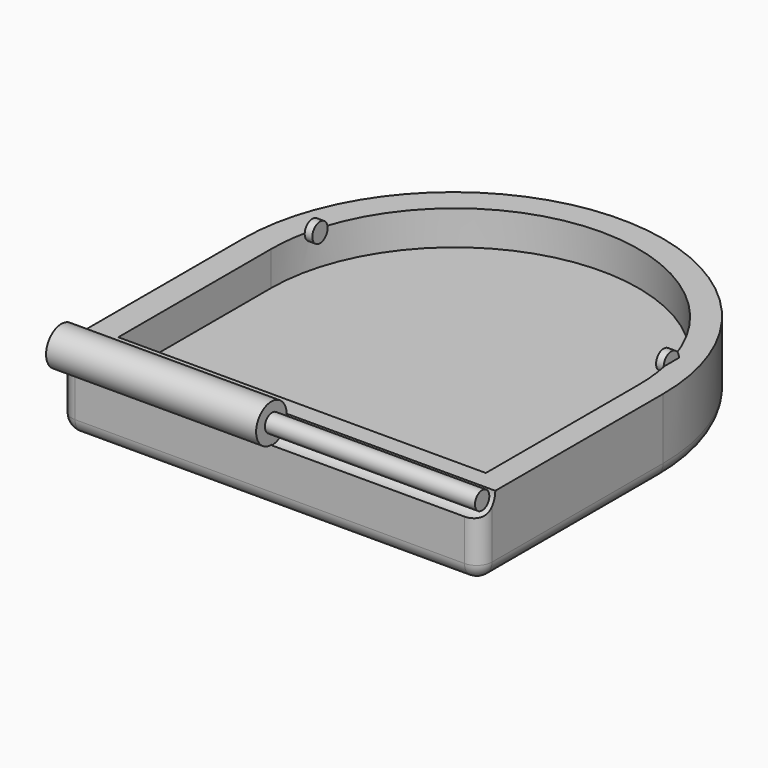
from build123d import *

# Parameters (mm, degrees)
F4_DEPTH       = 25.4
F1_R           = 6.35
F5_DEPTH       = 69.85
F3_R           = 6.604
F6_DEPTH       = 69.85
F7_R           = 5.07999
F2_R           = 2.9845
F8_DEPTH       = 69.85
F10_DEPTH      = 11.43
F12_DEPTH      = 25.4
F12_DEPTH_BACK = 25.4
F13_R          = 3.175
F14_DEPTH      = 59.69
F14_DEPTH_BACK = 59.69
F15_R          = 3.1877
F16_DEPTH      = 57.15
F16_DEPTH_BACK = 57.15


# Not quite as in the source:
# - a fillet or chamfer is up to 0.001 mm smaller than in the source, because OpenCascade refuses the exact size


with BuildPart() as f4:
    # F0 (on Top) → F4 (new body)
    with BuildSketch(Plane.XY):
        with BuildLine():
            Line((69.1548068551, -76.2), (69.1548068551, 0))
            ThreePointArc((69.1548068551, 0), (-0.6951931449, 69.85), (-70.5451931449, 0))
            Line((-70.5451931449, 0), (-70.5451931449, -76.2))
            Line((-70.5451931449, -76.2), (69.1548068551, -76.2))
        make_face()
    extrude(amount=-F4_DEPTH)

    # F1 (on Right) → F5 (join)
    with BuildSketch(Plane.YZ):
        with Locations((-76.4005258679, 0)):
            Circle(F1_R)
    extrude(amount=-F5_DEPTH)

    # F3 (on Right) → F6 (cut)
    with BuildSketch(Plane.YZ):
        with Locations((-76.365634799, 0)):
            Circle(F3_R)
    extrude(amount=F6_DEPTH, mode=Mode.SUBTRACT)

    # F7 (radius 5.08 in the source; OpenCascade refuses exactly that, so slightly less here)
    f7_edges = [f4.edges().sort_by_distance(p)[0] for p in [
        (-0.695193, -76.2, -25.4),
        (-70.545193, -38.1, -25.4),
        (-70.545193, -76.2, -12.7),
        (69.154807, -76.2, -16.000961),
    ]]
    fillet(f7_edges, radius=F7_R)

    # F2 (on Right) → F8 (join)
    with BuildSketch(Plane.YZ):
        with Locations((-76.0997384787, 0)):
            Circle(F2_R)
    extrude(amount=F8_DEPTH)

    # F9 (on Top) → F10 (cut)
    with BuildSketch(Plane.XY):
        with BuildLine():
            Line((60.994354069, -63.5), (60.994354069, 0))
            ThreePointArc((60.994354069, 0), (-0.118045931, 61.1124), (-61.230445931, 0))
            Line((-61.230445931, 0), (-61.230445931, -63.5))
            Line((-61.230445931, -63.5), (60.994354069, -63.5))
        make_face()
    extrude(amount=-F10_DEPTH, mode=Mode.SUBTRACT)

    # F11 (on Right) → F12 (cut, two sides)
    with BuildSketch(Plane.YZ) as f12_sk:
        Polygon((71.3768934982, -16.6989553797), (69.8592278852, 0), (69.8592278852, -4.7290348448), (65.7952278852, -4.7290348448), align=None)
    extrude(amount=-F12_DEPTH, mode=Mode.SUBTRACT)
    extrude(f12_sk.sketch, amount=F12_DEPTH_BACK, mode=Mode.SUBTRACT)

    # F13 (on Right) → F14 (join, two sides)
    with BuildSketch(Plane.YZ) as f14_sk:
        with Locations((15.24, 0)):
            Circle(F13_R)
    extrude(amount=F14_DEPTH)
    extrude(f14_sk.sketch, amount=-F14_DEPTH_BACK)

    # F15 (on Right) → F16 (cut, two sides)
    with BuildSketch(Plane.YZ) as f16_sk:
        with Locations((15.24, 0)):
            Circle(F15_R)
    extrude(amount=-F16_DEPTH, mode=Mode.SUBTRACT)
    extrude(f16_sk.sketch, amount=F16_DEPTH_BACK, mode=Mode.SUBTRACT)


solid = f4.part
